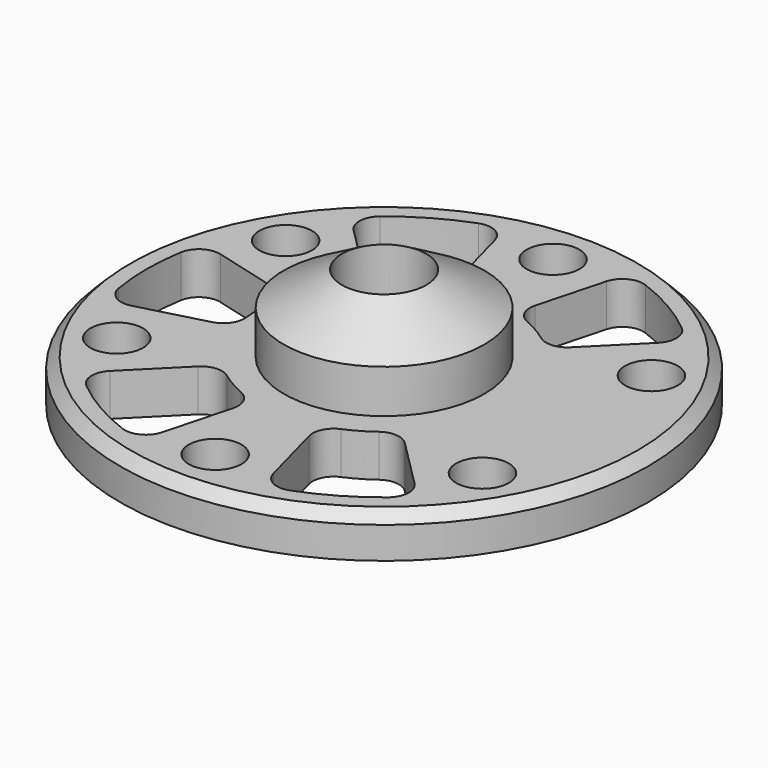
from build123d import *

# Parameters (mm, degrees)
F3_D            = 12.7
F3_COPIES_COUNT = 6
F5_DEPTH        = 10.161
F5_COPIES_COUNT = 5
F5_COPIES_ANGLE = 240
F6_R            = 5.08
F7_SIZE         = 2.54


# Not quite as in the source:
# - a pattern or mirror of a feature is missing from the dataset's text; its kind, count and spacing are read off the source's solid


with BuildPart() as f1:
    # F0 (on Front) → F1 (revolve)
    with BuildSketch(Plane.XZ):
        Polygon((10.16, 0), (63.5, 0), (63.5, 10.16), (24.13, 10.16), (24.13, 20.6138496578), (10.16, 28.6794329184), align=None)
    revolve(axis=Axis((0, 0, 9.6584064886), (0, 0, 1)))

    # F3 (through all)
    with Locations(Plane.XY.offset(10.16)):
        with Locations((0, 50.8)):
            f3 = Hole(F3_D / 2)

    # F3_copies: F3 ×6 about axis
    f3_copies_axis = Axis((0, 0, 0), (0, 0, 1))
    for i in range(1, F3_COPIES_COUNT):
        add(f3.rotate(f3_copies_axis, i * 360 / F3_COPIES_COUNT), mode=Mode.SUBTRACT)

    # F4 (on face) → F5 (cut, through all)
    with BuildSketch(Plane.XY.offset(10.16)):
        with BuildLine():
            ThreePointArc((7.8888044947, 29.4414191853), (15.24, 26.3964543073), (21.5526146906, 21.5526146906))
            Line((21.5526146906, 21.5526146906), (40.4111525448, 40.4111525448))
            ThreePointArc((40.4111525448, 40.4111525448), (28.575, 49.4933518263), (14.7915084276, 55.2026609724))
            Line((14.7915084276, 55.2026609724), (7.8888044947, 29.4414191853))
        make_face()
    f5 = extrude(amount=-F5_DEPTH, mode=Mode.SUBTRACT)

    # F5_copies: F5 ×5 about axis
    f5_copies_axis = Axis((0, 0, 0), (0, 0, 1))
    for i in range(1, F5_COPIES_COUNT):
        add(f5.rotate(f5_copies_axis, i * F5_COPIES_ANGLE / (F5_COPIES_COUNT - 1)), mode=Mode.SUBTRACT)

    # F6
    f6_edges = [f1.edges().sort_by_distance(p)[0] for p in [
        (14.791508, 55.202661, 5.08),
        (7.888804, 29.441419, 5.08),
        (21.552615, 21.552615, 5.08),
        (40.411153, 40.411153, 5.08),
        (14.791508, -55.202661, 5.08),
        (7.888804, -29.441419, 5.08),
        (21.552615, -21.552615, 5.08),
        (40.411153, -40.411153, 5.08),
        (-40.411153, -40.411153, 5.08),
        (-21.552615, -21.552615, 5.08),
        (-14.791508, -55.202661, 5.08),
        (-7.888804, -29.441419, 5.08),
        (-55.202661, 14.791508, 5.08),
        (-29.441419, 7.888804, 5.08),
        (-55.202661, -14.791508, 5.08),
        (-29.441419, -7.888804, 5.08),
        (-14.791508, 55.202661, 5.08),
        (-7.888804, 29.441419, 5.08),
        (-40.411153, 40.411153, 5.08),
        (-21.552615, 21.552615, 5.08),
    ]]
    fillet(f6_edges, radius=F6_R)

    # F7
    f7_edges = [f1.edges().sort_by_distance(p)[0] for p in [
        (-63.5, 0, 10.16),
    ]]
    chamfer(f7_edges, length=F7_SIZE)


solid = f1.part
